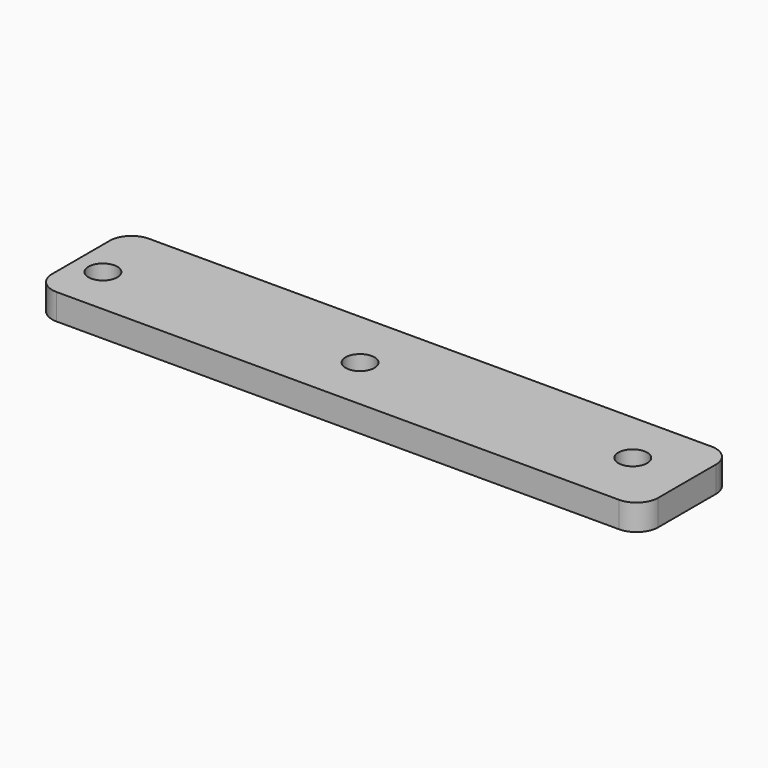
from build123d import *

# Parameters (mm, degrees)
F0_W     = 210
F0_H     = 40
F1_DEPTH = 9
F2_D     = 10
F3_R     = 7.5


with BuildPart() as f1:
    # F0 (on Top) → F1 (new body)
    with BuildSketch(Plane.XY):
        with Locations((0, 2.5)):
            Rectangle(F0_W, F0_H)
    extrude(amount=F1_DEPTH)

    # F2 (through all)
    with Locations(Plane(origin=(0, 0, 0), x_dir=(1, 0, 0), z_dir=(0, 0, -1))):
        with Locations((-95, 0.5), (-7.5, -1.5), (85, -4)):
            Hole(F2_D / 2)

    # F3
    f3_edges = [f1.edges().sort_by_distance(p)[0] for p in [
        (-105, 22.5, 4.5),
        (-105, -17.5, 4.5),
        (105, 22.5, 4.5),
        (105, -17.5, 4.5),
    ]]
    fillet(f3_edges, radius=F3_R)


solid = f1.part
